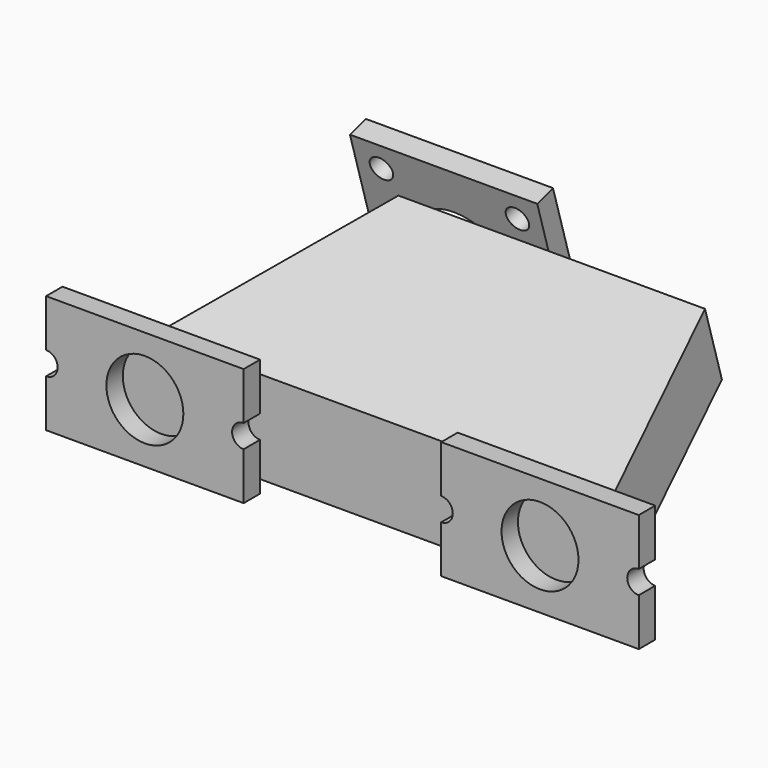
from build123d import *

# Parameters (mm, degrees)
F0_R     = 15
F1_DEPTH = 8
F4_W     = 73
F4_H     = 73
F4_R     = 4.4920969668
F4_R_2   = 19
F5_DEPTH = 8
F7_DEPTH = 97.5
F9_DEPTH = 78.5281878747


with BuildPart() as f1:
    # F0 (on Front) → F1 (new body)
    with BuildSketch(Plane.XZ):
        with BuildLine():
            Line((-38.5, 23), (-115.5, 23))
            Line((-115.5, 23), (-115.5, 4.5))
            ThreePointArc((-115.5, 4.5), (-111, 0), (-115.5, -4.5))
            Line((-115.5, -4.5), (-115.5, -23))
            Line((-115.5, -23), (-38.5, -23))
            Line((-38.5, -23), (-38.5, -4.5))
            ThreePointArc((-38.5, -4.5), (-43, 0), (-38.5, 4.5))
            Line((-38.5, 4.5), (-38.5, 23))
        make_face()
        with Locations((-77, 0)):
            Circle(F0_R, mode=Mode.SUBTRACT)
    extrude(amount=-F1_DEPTH)


with BuildPart() as f1b:
    # F0 (on Front) → F1, piece 2 (new body)
    with BuildSketch(Plane.XZ):
        with BuildLine():
            Line((115.5, 23), (38.5, 23))
            Line((38.5, 23), (38.5, 4.5))
            ThreePointArc((38.5, 4.5), (43, 0), (38.5, -4.5))
            Line((38.5, -4.5), (38.5, -23))
            Line((38.5, -23), (115.5, -23))
            Line((115.5, -23), (115.5, -4.5))
            ThreePointArc((115.5, -4.5), (111, 0), (115.5, 4.5))
            Line((115.5, 4.5), (115.5, 23))
        make_face()
        with Locations((77, 0)):
            Circle(F0_R, mode=Mode.SUBTRACT)
    extrude(amount=-F1_DEPTH)


with BuildPart() as f5:
    # F4 (on face) → F5 (new body)
    with BuildSketch(Plane(origin=(0, 75.9350016642, 22.6372071705), x_dir=(-1, 0, 0), z_dir=(0, 0.9583225745, 0.2856883674))):
        with Locations((0, 30)):
            Rectangle(F4_W, F4_H)
        with Locations((-26.5, 3.5)):
            Circle(F4_R, mode=Mode.SUBTRACT)
        with Locations((26.5, 3.5)):
            Circle(F4_R, mode=Mode.SUBTRACT)
        with Locations((-26.5, 56.5)):
            Circle(F4_R, mode=Mode.SUBTRACT)
        with Locations((0, 30)):
            Circle(F4_R_2, mode=Mode.SUBTRACT)
        with Locations((26.5, 56.5)):
            Circle(F4_R, mode=Mode.SUBTRACT)
    extrude(amount=-F5_DEPTH)


with BuildPart() as f7:
    # F6 (on Right) → F7 (new body, symmetric)
    with BuildSketch(Plane.YZ):
        Polygon((62.9987630306, 38.0284166596), (54.7667194692, 65.6422577498), (8, 18), (8, -18), align=None)
    extrude(amount=F7_DEPTH, both=True)

    # F8 (on face) → F9 (cut, through all)
    with BuildSketch(Plane(origin=(0, -4.9242673194, 4.8337723525), x_dir=(1, 0, 0), z_dir=(0, -0.7136337229, 0.7005190287))):
        Polygon((-80, 18.4495592417), (-22, 85.209657904), (-97.5, 85.209657904), (-97.5, 18.4495592417), align=None)
    extrude(amount=-F9_DEPTH, mode=Mode.SUBTRACT)


solid = Compound([f1.part, f1b.part, f5.part, f7.part])
